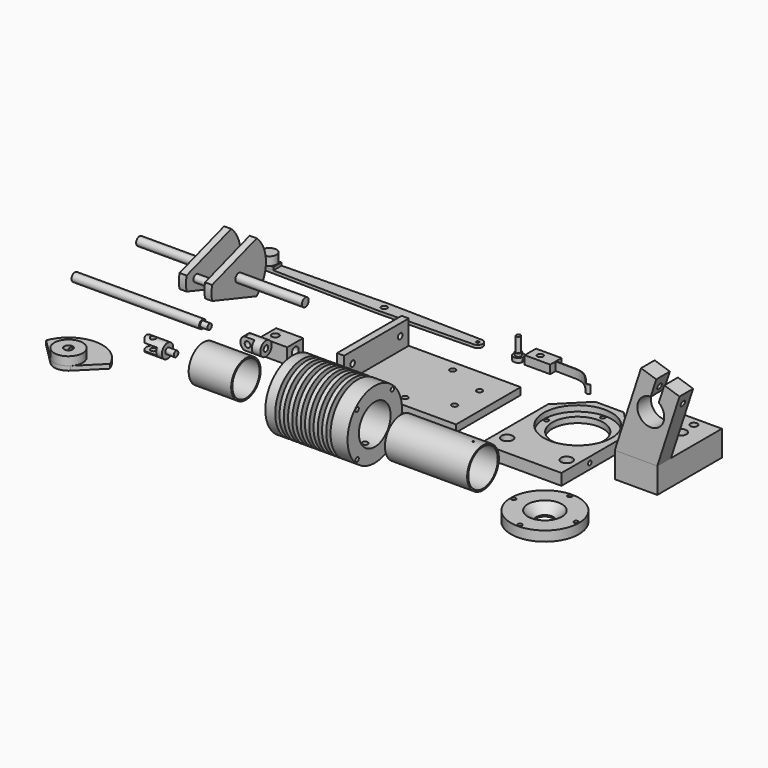
from build123d import *

# Parameters (mm, degrees)
F0_W           = 84
F0_H           = 57
F0_R           = 2
F1_DEPTH       = 5
F2_W           = 5
F2_H           = 57
F3_DEPTH       = 22
F4_R           = 2
F5_DEPTH       = 5
F6_R           = 2.1
F6_R_2         = 1.5
F6_R_3         = 18
F7_DEPTH       = 8
F8_R           = 4
F8_R_2         = 24
F9_DEPTH       = 4
F10_R          = 1.5
F11_DEPTH      = 10
F14_R          = 2
F15_DEPTH      = 14.61268
F16_R          = 1.5
F17_DEPTH      = 5
F18_R          = 1.5
F19_DEPTH      = 8
F20_W          = 58
F20_H          = 1
F22_R          = 0.5
F23_DEPTH      = 25
F24_R          = 24
F24_R_2        = 1.5
F24_R_3        = 6
F25_DEPTH      = 7
F26_SIZE       = 6
F27_W          = 30
F27_H          = 57
F28_DEPTH      = 18
F30_DEPTH      = 12
F31_R          = 4.5
F32_DEPTH      = 6
F33_R          = 2.5
F34_DEPTH      = 25
F35_R          = 4
F36_DEPTH      = 5
F37_R          = 2
F38_DEPTH      = 23.5316954889
F39_R          = 4
F40_DEPTH      = 5
F41_R          = 2.25
F42_DEPTH      = 25
F48_DEPTH      = 24.001000101
F48_DEPTH_BACK = 25
F49_W          = 16.0808475122
F49_H          = 19.4977000356
F50_DEPTH      = 2.5
F50_DEPTH_BACK = 2.5
F51_R          = 2
F52_DEPTH      = 53.0643909777
F52_DEPTH_BACK = 24.001000101
F55_W          = 10
F55_H          = 2.5
F56_DEPTH      = 434
F56_DEPTH_BACK = 25
F57_R          = 2
F58_DEPTH      = 5
F62_DEPTH      = 11
F63_R          = 3
F64_DEPTH      = 9
F65_W          = 14
F65_H          = 11
F65_R          = 1
F66_DEPTH      = 5
F67_R          = 2.5
F68_DEPTH      = 11
F69_R          = 1
F70_DEPTH      = 10
F73_R          = 2.5
F74_DEPTH      = 18
F76_DEPTH      = 23
F77_R          = 3
F78_DEPTH      = 3
F79_R          = 10
F79_R_2        = 3
F80_DEPTH      = 6
F82_W          = 2
F82_H          = 12.5130755996
F84_R          = 1.5
F84_R_2        = 2
F84_R_3        = 1
F85_DEPTH      = 2
F86_R          = 1.5
F87_DEPTH      = 2
F88_R          = 5
F89_DEPTH      = 6
F90_R          = 1.5
F91_DEPTH      = 5
F92_R          = 3.5
F93_DEPTH      = 3
F94_R          = 2
F95_DEPTH      = 2.1
F96_R          = 1.5
F97_DEPTH      = 10
F98_W          = 10
F98_H          = 1.5
F99_DEPTH      = 1.5
F100_R         = 2
F101_DEPTH     = 6


# Not quite as in the source:
# - an extrude ends at something that could not be found from the text; its depth is read off the source's solid
# - the dataset's text gives a spline's control points without its knots; the knots are read off the source's solid


with BuildPart() as f1:
    # F0 (on Top) → F1 (new body)
    with BuildSketch(Plane.XY):
        Rectangle(F0_W, F0_H)
        with Locations((0, -21)):
            Circle(F0_R, mode=Mode.SUBTRACT)
        with Locations((27, -11)):
            Circle(F0_R, mode=Mode.SUBTRACT)
        with Locations((27, 11)):
            Circle(F0_R, mode=Mode.SUBTRACT)
        with Locations((0, 21)):
            Circle(F0_R, mode=Mode.SUBTRACT)
    extrude(amount=F1_DEPTH)

    # F2 (on face) → F3 (join)
    with BuildSketch(Plane(origin=(0, 0, 0), x_dir=(1, 0, 0), z_dir=(0, 0, -1))):
        with Locations((-39.5, 0)):
            Rectangle(F2_W, F2_H)
    extrude(amount=-F3_DEPTH)

    # F4 (on face) → F5 (cut, through all)
    with BuildSketch(Plane(origin=(-42, 0, 0), x_dir=(0, -1, 0), z_dir=(-1, 0, 0))):
        with Locations((-21, 14)):
            Circle(F4_R)
        with Locations((21, 14)):
            Circle(F4_R)
    extrude(amount=-F5_DEPTH, mode=Mode.SUBTRACT)


with BuildPart() as f7:
    # F6 (on Top) → F7 (new body)
    with BuildSketch(Plane.XY):
        Polygon((70.1228168673, 17.5377150786), (70.1228168673, -41.9622849214), (127.1228168673, -41.9622849214), (127.1228168673, 17.5377150786), (108.6228168673, 36.0377150786), (88.6228168673, 36.0377150786), align=None)
        with Locations((77.6228168673, -27.9622849214)):
            Circle(F6_R, mode=Mode.SUBTRACT)
        with Locations((119.6228168673, -27.9622849214)):
            Circle(F6_R, mode=Mode.SUBTRACT)
        with Locations((98.6228168673, -13.9622849214)):
            Circle(F6_R_2, mode=Mode.SUBTRACT)
        with Locations((76.6228168673, 8.0377150786)):
            Circle(F6_R_2, mode=Mode.SUBTRACT)
        with Locations((98.6228168673, 8.0377150786)):
            Circle(F6_R_3, mode=Mode.SUBTRACT)
        with Locations((120.6228168673, 8.0377150786)):
            Circle(F6_R_2, mode=Mode.SUBTRACT)
        with Locations((98.6228168673, 30.0377150786)):
            Circle(F6_R_2, mode=Mode.SUBTRACT)
    extrude(amount=F7_DEPTH)

    # F8 (on face) → F9 (cut)
    with BuildSketch(Plane.XY.offset(8)):
        with Locations((77.6228168673, -27.9622849214)):
            Circle(F8_R)
        with Locations((119.6228168673, -27.9622849214)):
            Circle(F8_R)
        with Locations((98.6228168673, 8.0377150786)):
            Circle(F8_R_2)
    extrude(amount=-F9_DEPTH, mode=Mode.SUBTRACT)

    # F10 (on face) → F11 (cut)
    with BuildSketch(Plane.YZ.offset(127.1228168673)):
        with Locations((-16.9622849214, 4)):
            Circle(F10_R)
    extrude(amount=-F11_DEPTH, mode=Mode.SUBTRACT)


with BuildPart() as f13:
    # F12 (on face) → F13 (revolve)
    with BuildSketch(Plane.XY.offset(22)):
        Polygon((-30.6072234139, -57.9740965962), (-30.6072234139, -67.9740965962), (27.3927765861, -67.9740965962), (27.3927765861, -57.9740965962), (15.3927765861, -57.9740965962), (15.3927765861, -63.9740965962), (12.3927765861, -63.9740965962), (12.3927765861, -57.9740965962), (9.3927765861, -57.9740965962), (9.3927765861, -63.9740965962), (6.3927765861, -63.9740965962), (6.3927765861, -57.9740965962), (3.3927765861, -57.9740965962), (3.3927765861, -63.9740965962), (0.3927765861, -63.9740965962), (0.3927765861, -57.9740965962), (-2.6072234139, -57.9740965962), (-2.6072234139, -63.9740965962), (-5.6072234139, -63.9740965962), (-5.6072234139, -57.9740965962), (-8.6072234139, -57.9740965962), (-8.6072234139, -63.9740965962), (-11.6072234139, -63.9740965962), (-11.6072234139, -57.9740965962), (-14.6072234139, -57.9740965962), (-14.6072234139, -63.9740965962), (-17.6072234139, -63.9740965962), (-17.6072234139, -57.9740965962), (-20.6072234139, -57.9740965962), (-20.6072234139, -63.9740965962), (-23.6072234139, -63.9740965962), (-23.6072234139, -57.9740965962), align=None)
    revolve(axis=Axis((-1.6072234139, -81.9740965962, 22), (1, 0, 0)))

    # F14 (on Top) → F15 (cut, symmetric)
    with BuildSketch(Plane.XY):
        with Locations((20.3927765861, -81.9740965962)):
            Circle(F14_R)
    extrude(amount=F15_DEPTH, both=True, mode=Mode.SUBTRACT)

    # F16 (on face) → F17 (cut)
    with BuildSketch(Plane(origin=(-30.6072234139, 0, 0), x_dir=(0, -1, 0), z_dir=(-1, 0, 0))):
        with Locations((59.9740965962, 22)):
            Circle(F16_R)
        with Locations((103.9740965962, 22)):
            Circle(F16_R)
        with Locations((81.9740965962, 44)):
            Circle(F16_R)
        with Locations((81.9740965962, 0)):
            Circle(F16_R)
    extrude(amount=-F17_DEPTH, mode=Mode.SUBTRACT)

    # F18 (on face) → F19 (cut)
    with BuildSketch(Plane.YZ.offset(27.3927765861)):
        with Locations((-66.4177474101, 37.5563491861)):
            Circle(F18_R)
        with Locations((-66.4177474101, 6.4436508139)):
            Circle(F18_R)
        with Locations((-97.5304457823, 37.5563491861)):
            Circle(F18_R)
        with Locations((-97.5304457823, 6.4436508139)):
            Circle(F18_R)
    extrude(amount=-F19_DEPTH, mode=Mode.SUBTRACT)


with BuildPart() as f21:
    # F20 (on face) → F21 (revolve)
    with BuildSketch(Plane.XY.offset(22)):
        with Locations((77.2288471398, -71.5016102195)):
            Rectangle(F20_W, F20_H)
    revolve(axis=Axis((77.2288471398, -85.0016102195, 22), (-1, 0, 0)))

    # F22 (on face) → F23 (cut)
    with BuildSketch(Plane.XY.offset(22)):
        with Locations((99.2288471398, -85.0016102195)):
            Circle(F22_R)
    extrude(amount=F23_DEPTH, mode=Mode.SUBTRACT)


with BuildPart() as f25:
    # F24 (on Top) → F25 (new body)
    with BuildSketch(Plane.XY):
        with Locations((146.6991752386, -81.0055807233)):
            Circle(F24_R)
        with Locations((146.6991752386, -103.0055807233)):
            Circle(F24_R_2, mode=Mode.SUBTRACT)
        with Locations((168.6991752386, -81.0055807233)):
            Circle(F24_R_2, mode=Mode.SUBTRACT)
        with Locations((124.6991752386, -81.0055807233)):
            Circle(F24_R_2, mode=Mode.SUBTRACT)
        with Locations((146.6991752386, -81.0055807233)):
            Circle(F24_R_3, mode=Mode.SUBTRACT)
        with Locations((146.6991752386, -59.0055807233)):
            Circle(F24_R_2, mode=Mode.SUBTRACT)
    extrude(amount=F25_DEPTH)

    # F26
    f26_edges = [f25.edges().sort_by_distance(p)[0] for p in [
        (140.699175, -81.005581, 7),
    ]]
    chamfer(f26_edges, length=F26_SIZE)


with BuildPart() as f28:
    # F27 (on Top) → F28 (new body)
    with BuildSketch(Plane.XY):
        with Locations((160.1620242, 11.0399529512)):
            Rectangle(F27_W, F27_H)
    extrude(amount=F28_DEPTH)

    # F31 (on face) → F32 (cut)
    with BuildSketch(Plane(origin=(0, 0, 0), x_dir=(1, 0, 0), z_dir=(0, 0, -1))):
        with Locations((160.1620242, -33.5399529512)):
            Circle(F31_R)
        with Locations((160.1620242, 11.4600470488)):
            Circle(F31_R)
    extrude(amount=-F32_DEPTH, mode=Mode.SUBTRACT)


with BuildPart() as f30:
    # F29 (on face) → F30 (new body)
    with BuildSketch(Plane.XZ.offset(17.4600470488)):
        with BuildLine():
            Line((163.7030438625, 75.0633909777), (145.1620242, 18))
            Line((145.1620242, 18), (175.1620242, 18))
            Line((175.1620242, 18), (190.8382987781, 66.2466121933))
            Line((190.8382987781, 66.2466121933), (180.1238408692, 69.7279506024))
            Line((180.1238408692, 69.7279506024), (176.1980655738, 57.6456566053))
            ThreePointArc((176.1980655738, 57.6456566053), (167.6237930329, 40.9649630952), (170.4917264761, 59.4997585715))
            Line((170.4917264761, 59.4997585715), (174.4175017714, 71.5820525686))
            Line((174.4175017714, 71.5820525686), (163.7030438625, 75.0633909777))
        make_face()
    extrude(amount=-F30_DEPTH)


with BuildPart() as f34_tool:
    # F33 (on face) → F34 (new body)
    with BuildSketch(Plane(origin=(0, 0, 6), x_dir=(1, 0, 0), z_dir=(0, 0, -1))):
        with Locations((160.1620242, -33.5399529512)):
            Circle(F33_R)
        with Locations((160.1620242, 11.4600470488)):
            Circle(F33_R)
    extrude(amount=-F34_DEPTH)


with BuildPart() as f28_1:
    add(f28.part)

    # F34: cut by f34_tool
    add(f34_tool.part, mode=Mode.SUBTRACT)

    # F39 (on face) → F40 (cut)
    with BuildSketch(Plane.XY.offset(18)):
        with Locations((160.1620242, 0.0399529512)):
            Circle(F39_R)
        with Locations((160.1620242, 22.0399529512)):
            Circle(F39_R)
    extrude(amount=-F40_DEPTH, mode=Mode.SUBTRACT)

    # F41 (on face) → F42 (cut)
    with BuildSketch(Plane.XY.offset(13)):
        with Locations((160.1620242, 0.0399529512)):
            Circle(F41_R)
        with Locations((160.1620242, 22.0399529512)):
            Circle(F41_R)
    extrude(amount=-F42_DEPTH, mode=Mode.SUBTRACT)


with BuildPart() as f30_1:
    add(f30.part)

    # F34: cut by f34_tool
    add(f34_tool.part, mode=Mode.SUBTRACT)

    # F35 (on face) → F36 (cut)
    with BuildSketch(Plane(origin=(126.0102170872, 0, -40.9432014582), x_dir=(0, -1, 0), z_dir=(-0.9510565163, 0, 0.3090169944))):
        with Locations((11.4600470488, 113.976549709)):
            Circle(F35_R)
    extrude(amount=-F36_DEPTH, mode=Mode.SUBTRACT)

    # F37 (on face) → F38 (cut, through all)
    with BuildSketch(Plane(origin=(130.7654996686, 0, -42.4882864301), x_dir=(0, -1, 0), z_dir=(-0.9510565163, 0, 0.3090169944))):
        with Locations((11.4600470488, 113.976549709)):
            Circle(F37_R)
    extrude(amount=-F38_DEPTH, mode=Mode.SUBTRACT)


with BuildPart() as f44:
    # F43 (on face) → F44 (revolve)
    with BuildSketch(Plane.XY.offset(22)):
        Polygon((-61.9552821589, -71.9084982872), (-61.9552821589, -70.9084982872), (-91.9552821589, -70.9084982872), (-91.9552821589, -81.9084982872), (-85.9552821589, -81.9084982872), (-85.9552821589, -71.9084982872), align=None)
    revolve(axis=Axis((-76.9552821589, -83.9084982872, 22), (-1, 0, 0)))


with BuildPart() as f46:
    # F45 (on face) → F46 (revolve)
    with BuildSketch(Plane.XY.offset(22)):
        Polygon((-110.6047921076, -84.6925973892), (-131.6047921076, -84.6925973892), (-131.6047921076, -89.6925973892), (-116.6047921076, -89.6925973892), (-116.6047921076, -86.6925973892), (-110.6047921076, -86.6925973892), align=None)
    revolve(axis=Axis((-121.1047921076, -84.6925973892, 22), (1, 0, 0)))

    # F47 (on face) → F48 (cut, two sides)
    with BuildSketch(Plane.XY.offset(22)) as f48_sk:
        with BuildLine():
            ThreePointArc((-126.6047921076, -89.6925973892), (-131.6047921076, -84.6925973892), (-126.6047921076, -79.6925973892))
            Line((-126.6047921076, -79.6925973892), (-135.0083202124, -79.6925973892))
            Line((-135.0083202124, -79.6925973892), (-135.0083202124, -89.6925973892))
            Line((-135.0083202124, -89.6925973892), (-126.6047921076, -89.6925973892))
        make_face()
    extrude(amount=-F48_DEPTH, mode=Mode.SUBTRACT)
    extrude(f48_sk.sketch, amount=F48_DEPTH_BACK, mode=Mode.SUBTRACT)

    # F49 (on face) → F50 (cut, two sides)
    with BuildSketch(Plane.XY.offset(22)) as f50_sk:
        with Locations((-128.6452158637, -84.9742926657)):
            Rectangle(F49_W, F49_H)
    extrude(amount=F50_DEPTH, mode=Mode.SUBTRACT)
    extrude(f50_sk.sketch, amount=-F50_DEPTH_BACK, mode=Mode.SUBTRACT)

    # F51 (on face) → F52 (cut, two sides)
    with BuildSketch(Plane.XY.offset(22)) as f52_sk:
        with Locations((-126.6047921076, -84.6925973892)):
            Circle(F51_R)
    extrude(amount=F52_DEPTH, mode=Mode.SUBTRACT)
    extrude(f52_sk.sketch, amount=-F52_DEPTH_BACK, mode=Mode.SUBTRACT)


with BuildPart() as f54:
    # F53 (on face) → F54 (revolve)
    with BuildSketch(Plane.XY.offset(22)):
        Polygon((-75.9198864996, -43.7728373113), (-91.9198864996, -43.7728373113), (-91.9198864996, -48.7728373113), (-80.9198864996, -48.7728373113), (-80.9198864996, -46.7728373113), (-75.9198864996, -46.7728373113), align=None)
    revolve(axis=Axis((-86.4198864996, -48.7728373113, 22), (1, 0, 0)))

    # F55 (on face) → F56 (cut, two sides)
    with BuildSketch(Plane.XY.offset(22)) as f56_sk:
        with Locations((-86.9198864996, -45.0228373113)):
            Rectangle(F55_W, F55_H)
        with Locations((-86.9198864996, -52.5228373113)):
            Rectangle(F55_W, F55_H)
    extrude(amount=-F56_DEPTH, mode=Mode.SUBTRACT)
    extrude(f56_sk.sketch, amount=F56_DEPTH_BACK, mode=Mode.SUBTRACT)

    # F57 (on face) → F58 (cut, through all)
    with BuildSketch(Plane(origin=(0, -46.2728373113, 0), x_dir=(-1, 0, 0), z_dir=(0, 1, 0))):
        with BuildLine():
            ThreePointArc((86.9198864996, 27), (91.9198864996, 22), (86.9198864996, 17))
            Line((86.9198864996, 17), (95.1001867652, 17))
            Line((95.1001867652, 17), (95.1001867652, 27))
            Line((95.1001867652, 27), (86.9198864996, 27))
        make_face()
        with Locations((86.9198864996, 22)):
            Circle(F57_R)
    extrude(amount=-F58_DEPTH, mode=Mode.SUBTRACT)


with BuildPart() as f60:
    # F59 (on face) → F60 (revolve)
    with BuildSketch(Plane.XY.offset(22)):
        Polygon((-116.502759822, -49.7975535003), (-116.502759822, -47.7975535003), (-211.502759822, -47.7975535003), (-211.502759822, -50.7975535003), (-121.502759822, -50.7975535003), (-121.502759822, -49.7975535003), align=None)
    revolve(axis=Axis((-164.002759822, -47.7975535003, 22), (-1, 0, 0)))


with BuildPart() as f62:
    # F61 (on Top) → F62 (new body)
    with BuildSketch(Plane.XY):
        with BuildLine():
            Line((-94.9450552166, -23.7235993746), (-80.9450552166, -23.7235993746))
            Line((-80.9450552166, -23.7235993746), (-80.9450552166, -9.7235993746))
            Line((-80.9450552166, -9.7235993746), (-94.9450552166, -9.7235993746))
            Line((-94.9450552166, -9.7235993746), (-94.9450552166, -14.2235993746))
            ThreePointArc((-94.9450552166, -14.2235993746), (-92.4450552166, -16.7235993746), (-94.9450552166, -19.2235993746))
            Line((-94.9450552166, -19.2235993746), (-94.9450552166, -23.7235993746))
        make_face()
    extrude(amount=F62_DEPTH)

    # F63 (on face) → F64 (cut)
    with BuildSketch(Plane.YZ.offset(-80.9450552166)):
        with Locations((-16.7235993746, 5.5)):
            Circle(F63_R)
    extrude(amount=-F64_DEPTH, mode=Mode.SUBTRACT)

    # F69 (on face) → F70 (cut)
    with BuildSketch(Plane(origin=(-94.9450552166, 0, 0), x_dir=(0, -1, 0), z_dir=(-1, 0, 0))):
        with Locations((21.4735993746, 5.5)):
            Circle(F69_R)
        with Locations((11.9735993746, 5.5)):
            Circle(F69_R)
    extrude(amount=-F70_DEPTH, mode=Mode.SUBTRACT)


with BuildPart() as f66:
    # F65 (on face) → F66 (new body)
    with BuildSketch(Plane(origin=(-94.9450552166, 0, 0), x_dir=(0, -1, 0), z_dir=(-1, 0, 0))):
        with Locations((16.7235993746, 5.5)):
            Rectangle(F65_W, F65_H)
        with Locations((11.9735993746, 5.5)):
            Circle(F65_R, mode=Mode.SUBTRACT)
        with Locations((21.4735993746, 5.5)):
            Circle(F65_R, mode=Mode.SUBTRACT)
    extrude(amount=F66_DEPTH)

    # F67 (on face) → F68 (cut, through all)
    with BuildSketch(Plane.XY.offset(11)):
        with Locations((-94.9450552166, -16.7235993746)):
            Circle(F67_R)
    extrude(amount=-F68_DEPTH, mode=Mode.SUBTRACT)


with BuildPart() as f72:
    # F71 (on face) → F72 (revolve)
    with BuildSketch(Plane.XY.offset(22)):
        Polygon((-93.5209851265, 7.9587362707), (-145.5209851265, 7.9587362707), (-145.5209851265, -16.0412637293), (-140.5209851265, -16.0412637293), (-140.5209851265, 4.9587362707), (-93.5209851265, 4.9587362707), align=None)
    revolve(axis=Axis((-119.5209851265, 7.9587362707, 22), (1, 0, 0)))



with BuildPart() as f72b:
    # F71 (on face) → F72, piece 2 (revolve)
    with BuildSketch(Plane.XY.offset(22)):
        Polygon((-163.5209851265, -16.0412637293), (-158.5209851265, -16.0412637293), (-158.5209851265, 7.9587362707), (-210.5209851265, 7.9587362707), (-210.5209851265, 4.9587362707), (-163.5209851265, 4.9587362707), align=None)
    revolve(axis=Axis((-119.5209851265, 7.9587362707, 22), (1, 0, 0)))


with BuildPart() as f72_1:
    add(f72.part)

    add(f72b.part)  # F74 merges F72b
    # F73 (on face) → F74 (join, through all)
    with BuildSketch(Plane(origin=(-163.5209851265, 0, 0), x_dir=(0, -1, 0), z_dir=(-1, 0, 0))):
        with Locations((7.0412637293, 22)):
            Circle(F73_R)
    extrude(amount=-F74_DEPTH)

    # F75 (on face) → F76 (cut, through all)
    with BuildSketch(Plane(origin=(-163.5209851265, 0, 0), x_dir=(0, -1, 0), z_dir=(-1, 0, 0))):
        Polygon((15.5146529179, -5.5542048228), (15.5146529179, 17), (-23.8332441371, 4), (-23.8332441371, -5.5542048228), align=None)
        Polygon((-23.8332441371, 40), (15.5146529179, 27), (15.5146529179, 49.5542048228), (-23.8332441371, 49.5542048228), align=None)
    extrude(amount=-F76_DEPTH, mode=Mode.SUBTRACT)


with BuildPart() as f78:
    # F77 (on Top) → F78 (new body)
    with BuildSketch(Plane.XY):
        with BuildLine():
            Line((-169.9269427203, -103.6596482934), (-154.4965853534, -88.2355090458))
            ThreePointArc((-154.4965853534, -88.2355090458), (-176.9965853534, -72.58715559), (-199.4965853534, -88.2355090458))
            Line((-199.4965853534, -88.2355090458), (-184.0662279866, -103.6596482934))
            ThreePointArc((-184.0662279866, -103.6596482934), (-176.9965853534, -106.58715559), (-169.9269427203, -103.6596482934))
        make_face()
        with Locations((-176.9965853534, -96.58715559)):
            Circle(F77_R, mode=Mode.SUBTRACT)
    extrude(amount=F78_DEPTH)

    # F79 (on face) → F80 (join)
    with BuildSketch(Plane.XY.offset(3)):
        with Locations((-176.9965853534, -96.58715559)):
            Circle(F79_R)
        with Locations((-176.9965853534, -96.58715559)):
            Circle(F79_R_2, mode=Mode.SUBTRACT)
    extrude(amount=F80_DEPTH)

    # F82 (on offset) → F83 (revolve, cut)
    with BuildSketch(Plane.XY.offset(6)):
        with Locations((-175.9965853534, -90.3306177902)):
            Rectangle(F82_W, F82_H)
    revolve(axis=Axis((-176.9965853534, -90.3306177902, 6), (0, 1, 0)), mode=Mode.SUBTRACT)


with BuildPart() as f85:
    # F84 (on Top) → F85 (new body)
    with BuildSketch(Plane.XY):
        with BuildLine():
            Line((-79.7108555386, 65.2738681436), (-160.7756333471, 63.7732686401))
            ThreePointArc((-160.7756333471, 63.7732686401), (-164.2108555386, 60.2738681436), (-160.7756333471, 56.774467647))
            Line((-160.7756333471, 56.774467647), (-79.7108555386, 55.2738681436))
            Line((-79.7108555386, 55.2738681436), (-13.6313784545, 56.7747706323))
            ThreePointArc((-13.6313784545, 56.7747706323), (-10.2108555386, 60.2738681436), (-13.6313784545, 63.7729656548))
            Line((-13.6313784545, 63.7729656548), (-79.7108555386, 65.2738681436))
        make_face()
        with Locations((-160.7108555386, 60.2738681436)):
            Circle(F84_R, mode=Mode.SUBTRACT)
        with Locations((-79.7108555386, 60.2738681436)):
            Circle(F84_R_2, mode=Mode.SUBTRACT)
        with Locations((-13.7108555386, 60.2738681436)):
            Circle(F84_R_3, mode=Mode.SUBTRACT)
    extrude(amount=F85_DEPTH)

    # F86 (on face) → F87 (join)
    with BuildSketch(Plane.XY.offset(2)):
        with BuildLine():
            Line((-155.0315705785, 56.6681386349), (-155.0315705785, 63.8795976522))
            Line((-155.0315705785, 63.8795976522), (-160.7756333471, 63.7732686401))
            ThreePointArc((-160.7756333471, 63.7732686401), (-164.2108555386, 60.2738681436), (-160.7756333471, 56.774467647))
            Line((-160.7756333471, 56.774467647), (-155.0315705785, 56.6681386349))
        make_face()
        with Locations((-160.7108555386, 60.2738681436)):
            Circle(F86_R, mode=Mode.SUBTRACT)
    extrude(amount=F87_DEPTH)


with BuildPart() as f89:
    # F88 (on face) → F89 (new body)
    with BuildSketch(Plane.XY.offset(4)):
        with Locations((-160.7108555386, 60.2738681436)):
            Circle(F88_R)
    extrude(amount=F89_DEPTH)

    # F90 (on face) → F91 (join)
    with BuildSketch(Plane(origin=(0, 0, 4), x_dir=(1, 0, 0), z_dir=(0, 0, -1))):
        with Locations((-160.7108555386, -60.2738681436)):
            Circle(F90_R)
    extrude(amount=F91_DEPTH)


with BuildPart() as f93:
    # F92 (on Top) → F93 (new body)
    with BuildSketch(Plane.XY):
        with Locations((14.7544275969, 60.5189241469)):
            Circle(F92_R)
    extrude(amount=F93_DEPTH)

    # F94 (on face) → F95 (join)
    with BuildSketch(Plane.XY.offset(3)):
        with Locations((14.7544275969, 60.5189241469)):
            Circle(F94_R)
    extrude(amount=F95_DEPTH)

    # F96 (on face) → F97 (join)
    with BuildSketch(Plane.XY.offset(5.1)):
        with Locations((14.7544275969, 60.5189241469)):
            Circle(F96_R)
    extrude(amount=F97_DEPTH)

    # F98 (on face) → F99 (cut)
    with BuildSketch(Plane(origin=(0, 0, 0), x_dir=(1, 0, 0), z_dir=(0, 0, -1))):
        with Locations((14.7544275969, -60.5189241469)):
            Rectangle(F98_W, F98_H)
    extrude(amount=-F99_DEPTH, mode=Mode.SUBTRACT)


with BuildPart() as f101:
    # F100 (on Top) → F101 (new body)
    with BuildSketch(Plane.XY):
        with BuildLine():
            Line((39.0966013074, 63.3197225571), (39.0966013074, 68.1697225571))
            Line((39.0966013074, 68.1697225571), (21.0966013074, 68.1697225571))
            Line((21.0966013074, 68.1697225571), (21.0966013074, 58.1697225571))
            Line((21.0966013074, 58.1697225571), (39.0966013074, 58.1697225571))
            Line((39.0966013074, 58.1697225571), (39.0966013074, 63.019685613))
            add(Edge.make_bspline(
                [(39.0966013074, 63.0196856127), (39.8170344897, 63.0084050405), (41.5163646936, 63.0057561802), (44.5609808064, 63.02262594), (47.2756736278, 63.0218130582), (49.4097420981, 62.9928951659), (50.955153538, 62.952283952), (52.4102961474, 62.8879180438), (53.7344392941, 62.7953725263), (54.9374572251, 62.6674338517), (56.4049933856, 62.4395432499), (58.0253305007, 62.0291116121), (59.775256209, 61.2749061009), (61.4813650604, 60.1901135084), (62.838933747, 59.0551109262), (63.87093491, 58.0354344594), (64.6146537481, 57.222476582), (65.3220500201, 56.365327906), (66.0030879586, 55.4809495901), (66.669692886, 54.6283886692), (67.3353998002, 53.8586415485), (67.9046932996, 53.329136165), (68.383443283, 53.0004287134), (68.7577648866, 52.8103033304), (69.1543731783, 52.6878555145), (69.6915866458, 52.633324616), (70.3319375454, 52.7385368735), (70.97410521, 53.064568044), (71.2732370072, 53.3898503761), (71.3669696098, 53.584785677)],
                knots=[0.0001362079, 0.0001362079, 0.0001362079, 0.0001362079, 0.0625, 0.125, 0.1875, 0.21875, 0.25, 0.28125, 0.3125, 0.34375, 0.375, 0.4375, 0.5, 0.5625, 0.625, 0.65625, 0.6875, 0.71875, 0.75, 0.78125, 0.8125, 0.84375, 0.859375, 0.875, 0.890625, 0.90625, 0.9375, 0.96875, 1, 1, 1, 1], degree=3))
            Line((71.3669696098, 53.584785677), (71.0966013074, 53.7147894502))
            add(Edge.make_bspline(
                [(39.0966013074, 63.3197225571), (42.3855919461, 63.2679844268), (52.8895700746, 63.5412439918), (59.9169355021, 62.1604904948), (65.3066397838, 57.3928619389), (68.5454742559, 52.1523154859), (70.8589313943, 53.2205083276), (71.0966013074, 53.7147894502)],
                knots=[0, 0, 0, 0, 0.2862577113, 0.4981945524, 0.7051525004, 0.8884229192, 1, 1, 1, 1], degree=3))
        make_face()
        with Locations((28.0966013074, 63.1697225571)):
            Circle(F100_R, mode=Mode.SUBTRACT)
    extrude(amount=F101_DEPTH)


solid = Compound([f1.part, f7.part, f13.part, f21.part, f25.part, f28_1.part, f30_1.part, f44.part, f46.part, f54.part, f60.part, f62.part, f66.part, f72_1.part, f78.part, f85.part, f89.part, f93.part, f101.part])
